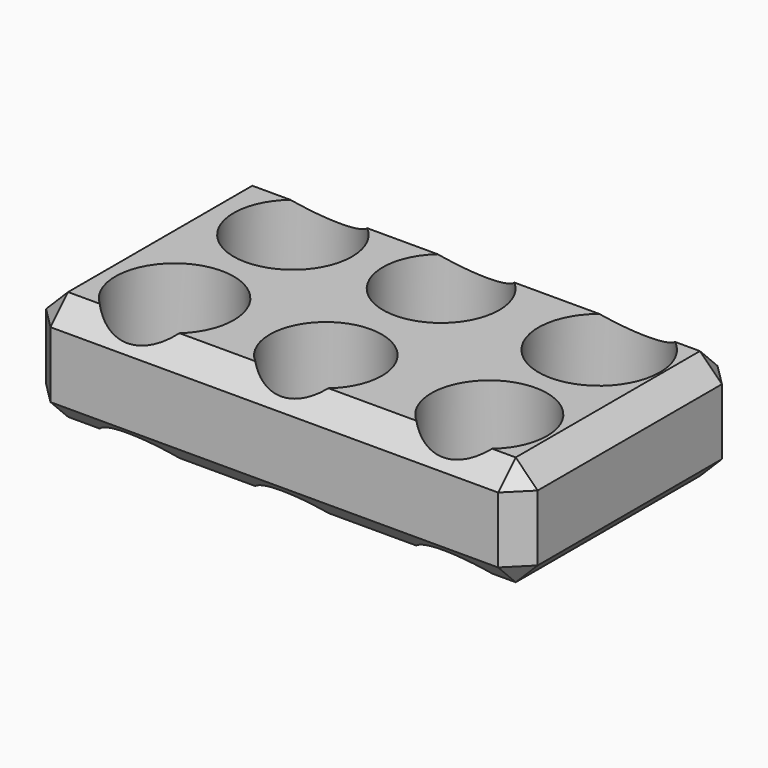
from build123d import *

# Parameters (mm, degrees)
F0_W         = 113.590836525
F0_H         = 63.365586102
F0_R         = 13.6776668511
F0_R_2       = 12.9483089266
F0_R_3       = 13.3718975465
F0_R_4       = 13.6714310258
F0_R_5       = 14.0406678545
F0_R_6       = 13.4346835475
F1_DEPTH     = 25.4
F2_W         = 109.635181725
F2_H         = 62.0416179299
F2_R         = 13.6776668511
F2_R_2       = 12.9483089266
F2_R_3       = 13.3718975465
F2_R_4       = 13.6714310258
F2_R_5       = 14.0406678545
F2_R_6       = 13.4346835475
F3_DEPTH     = 12.7
F4_T1_DEPTH  = 6.4524666085
F4_T3_DEPTH  = 6.4524666085
F4_T5_DEPTH  = 6.4524666085
F4_T7_DEPTH  = 6.4524666085
F4_T9_DEPTH  = 6.4524666085
F4_T11_DEPTH = 6.4524666085
F4_T13_DEPTH = 6.4524666085
F4_T15_DEPTH = 6.4524666085
F4_T17_DEPTH = 89.4938852597
F4_T19_DEPTH = 139.7191356827
F4_T21_DEPTH = 51.5282991577


# Not quite as in the source:
# - a fillet or chamfer that OpenCascade refuses, or shapes differently, is made with other operations: its cross-section is extruded or revolved along the edge and cut away or added


with BuildPart() as f1:
    # F0 (on Top) → F1 (new body)
    with BuildSketch(Plane.XY):
        Rectangle(F0_W, F0_H)
        with Locations((-35.1868793368, -16.4984129369)):
            Circle(F0_R, mode=Mode.SUBTRACT)
        with Locations((0, -16.790419817)):
            Circle(F0_R_2, mode=Mode.SUBTRACT)
        with Locations((37.5229418278, -16.4984129369)):
            Circle(F0_R_3, mode=Mode.SUBTRACT)
        with Locations((-34.0188518167, 16.2064060569)):
            Circle(F0_R_4, mode=Mode.SUBTRACT)
        with Locations((37.2309349477, 15.6223904341)):
            Circle(F0_R_5, mode=Mode.SUBTRACT)
        with Locations((0, 16.4984129369)):
            Circle(F0_R_6, mode=Mode.SUBTRACT)
    extrude(amount=F1_DEPTH)

    # F2 (on face) → F3 (join)
    with BuildSketch(Plane.XY):
        Rectangle(F2_W, F2_H)
        with Locations((-35.1868793368, -16.4984129369)):
            Circle(F2_R, mode=Mode.SUBTRACT)
        with Locations((0, -16.790419817)):
            Circle(F2_R_2, mode=Mode.SUBTRACT)
        with Locations((37.5229418278, -16.4984129369)):
            Circle(F2_R_3, mode=Mode.SUBTRACT)
        with Locations((-34.0188518167, 16.2064060569)):
            Circle(F2_R_4, mode=Mode.SUBTRACT)
        with Locations((37.2309349477, 15.6223904341)):
            Circle(F2_R_5, mode=Mode.SUBTRACT)
        with Locations((0, 16.4984129369)):
            Circle(F2_R_6, mode=Mode.SUBTRACT)
    extrude(amount=F3_DEPTH)

    # F4: chamfer of 5.08 on 12 edges, made by hand

    # F4_s2 → F4_t1 (cut)
    with BuildSketch(Plane(origin=(26.1060704378, -26.1060704378, -26.1060704378), x_dir=(0.7071067812, 0.7071067812, 0), z_dir=(0.5773502692, -0.5773502692, -0.5773502692))):
        Polygon((14.165205132, 38.1949798276), (17.7573075804, 31.9732758809), (21.3494100289, 38.1949798276), align=None)
    extrude(amount=F4_T1_DEPTH, mode=Mode.SUBTRACT)

    # F4_s4 → F4_t3 (cut)
    with BuildSketch(Plane(origin=(26.1060704378, 26.1060704378, -26.1060704378), x_dir=(-0.7071067812, 0.7071067812, 0), z_dir=(0.5773502692, 0.5773502692, -0.5773502692))):
        Polygon((-14.165205132, 38.1949798276), (-17.7573075804, 31.9732758809), (-21.3494100289, 38.1949798276), align=None)
    extrude(amount=F4_T3_DEPTH, mode=Mode.SUBTRACT)

    # F4_s6 → F4_t5 (cut)
    with BuildSketch(Plane(origin=(-26.1060704378, 26.1060704378, -26.1060704378), x_dir=(-0.7071067812, -0.7071067812, 0), z_dir=(-0.5773502692, 0.5773502692, -0.5773502692))):
        Polygon((14.165205132, 38.1949798276), (17.7573075804, 31.9732758809), (21.3494100289, 38.1949798276), align=None)
    extrude(amount=F4_T5_DEPTH, mode=Mode.SUBTRACT)

    # F4_s8 → F4_t7 (cut)
    with BuildSketch(Plane(origin=(-26.1060704378, -26.1060704378, -26.1060704378), x_dir=(0.7071067812, -0.7071067812, 0), z_dir=(-0.5773502692, -0.5773502692, -0.5773502692))):
        Polygon((-14.165205132, 38.1949798276), (-17.7573075804, 31.9732758809), (-21.3494100289, 38.1949798276), align=None)
    extrude(amount=F4_T7_DEPTH, mode=Mode.SUBTRACT)

    # F4_s10 → F4_t9 (cut)
    with BuildSketch(Plane(origin=(-34.5727371045, 34.5727371045, 34.5727371045), x_dir=(-0.7071067812, -0.7071067812, 0), z_dir=(-0.5773502692, 0.5773502692, 0.5773502692))):
        Polygon((14.165205132, -17.455966672), (17.7573075804, -11.2342627254), (21.3494100289, -17.455966672), align=None)
    extrude(amount=F4_T9_DEPTH, mode=Mode.SUBTRACT)

    # F4_s12 → F4_t11 (cut)
    with BuildSketch(Plane(origin=(34.5727371045, -34.5727371045, 34.5727371045), x_dir=(0.7071067812, 0.7071067812, 0), z_dir=(0.5773502692, -0.5773502692, 0.5773502692))):
        Polygon((14.165205132, -17.455966672), (17.7573075804, -11.2342627254), (21.3494100289, -17.455966672), align=None)
    extrude(amount=F4_T11_DEPTH, mode=Mode.SUBTRACT)

    # F4_s14 → F4_t13 (cut)
    with BuildSketch(Plane(origin=(34.5727371045, 34.5727371045, 34.5727371045), x_dir=(-0.7071067812, 0.7071067812, 0), z_dir=(0.5773502692, 0.5773502692, 0.5773502692))):
        Polygon((-14.165205132, -17.455966672), (-17.7573075804, -11.2342627254), (-21.3494100289, -17.455966672), align=None)
    extrude(amount=F4_T13_DEPTH, mode=Mode.SUBTRACT)

    # F4_s16 → F4_t15 (cut)
    with BuildSketch(Plane(origin=(-34.5727371045, -34.5727371045, 34.5727371045), x_dir=(0.7071067812, -0.7071067812, 0), z_dir=(-0.5773502692, -0.5773502692, 0.5773502692))):
        Polygon((-14.165205132, -17.455966672), (-17.7573075804, -11.2342627254), (-21.3494100289, -17.455966672), align=None)
    extrude(amount=F4_T15_DEPTH, mode=Mode.SUBTRACT)

    # F4_s18 → F4_t17 (cut)
    with BuildSketch(Plane.XZ.offset(-44.7469426299)):
        Polygon((51.7154182625, 0), (56.7954182625, 5.08), (56.7954182625, 0), align=None)
        Polygon((-51.7154182625, 0), (-56.7954182625, 5.08), (-56.7954182625, 0), align=None)
        Polygon((-51.7154182625, 25.4), (-56.7954182625, 20.32), (-56.7954182625, 25.4), align=None)
        Polygon((51.7154182625, 25.4), (56.7954182625, 20.32), (56.7954182625, 25.4), align=None)
    extrude(amount=F4_T17_DEPTH, mode=Mode.SUBTRACT)

    # F4_s20 → F4_t19 (cut)
    with BuildSketch(Plane.YZ.offset(-69.8595678413)):
        Polygon((31.682793051, 5.08), (26.602793051, 0), (31.682793051, 0), align=None)
        Polygon((-31.682793051, 5.08), (-26.602793051, 0), (-31.682793051, 0), align=None)
        Polygon((31.682793051, 20.32), (26.602793051, 25.4), (31.682793051, 25.4), align=None)
        Polygon((-26.602793051, 25.4), (-31.682793051, 20.32), (-31.682793051, 25.4), align=None)
    extrude(amount=F4_T19_DEPTH, mode=Mode.SUBTRACT)

    # F4_s22 → F4_t21 (cut)
    with BuildSketch(Plane.XY.offset(-13.0641495789)):
        Polygon((-51.7154182625, 31.682793051), (-56.7954182625, 26.602793051), (-56.7954182625, 31.682793051), align=None)
        Polygon((51.7154182625, -31.682793051), (56.7954182625, -26.602793051), (56.7954182625, -31.682793051), align=None)
        Polygon((-51.7154182625, -31.682793051), (-56.7954182625, -26.602793051), (-56.7954182625, -31.682793051), align=None)
        Polygon((51.7154182625, 31.682793051), (56.7954182625, 26.602793051), (56.7954182625, 31.682793051), align=None)
    extrude(amount=F4_T21_DEPTH, mode=Mode.SUBTRACT)


solid = f1.part
